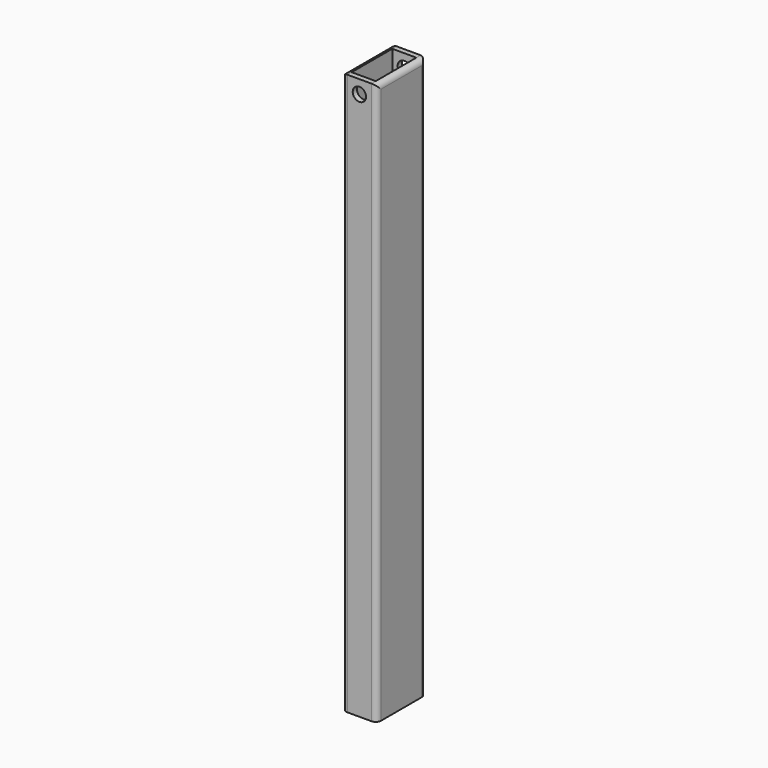
from build123d import *

# Parameters (mm, degrees)
F0_W     = 33.02
F0_H     = 533.4
F1_DEPTH = 58.42
F3_T     = -5.08
F4_D     = 12.7
F5_R     = 5.07999


# Not quite as in the source:
# - a fillet or chamfer is up to 0.001 mm smaller than in the source, because OpenCascade refuses the exact size


with BuildPart() as f1:
    # F0 (on Front) → F1 (new body)
    with BuildSketch(Plane.XZ):
        with Locations((16.51, -266.7)):
            Rectangle(F0_W, F0_H)
    extrude(amount=F1_DEPTH)

    # F3
    f3_openings = [f1.faces().sort_by_distance(p)[0] for p in [
        (16.51, -29.21, 0),
        (16.51, -29.21, -533.4),
    ]]
    offset(amount=F3_T, openings=f3_openings)

    # F4 (through all)
    with Locations(Plane.XZ.offset(58.42)):
        with Locations((16.51, -12.7)):
            Hole(F4_D / 2)

    # F5 (radius 5.08 in the source; OpenCascade refuses exactly that, so slightly less here)
    f5_edges = [f1.edges().sort_by_distance(p)[0] for p in [
        (0, -58.42, -266.7),
        (33.02, -58.42, -266.7),
        (33.02, 0, -266.7),
        (0, 0, -266.7),
        (33.02, -29.21, 0),
        (0, -29.21, 0),
    ]]
    fillet(f5_edges, radius=F5_R)


solid = f1.part
